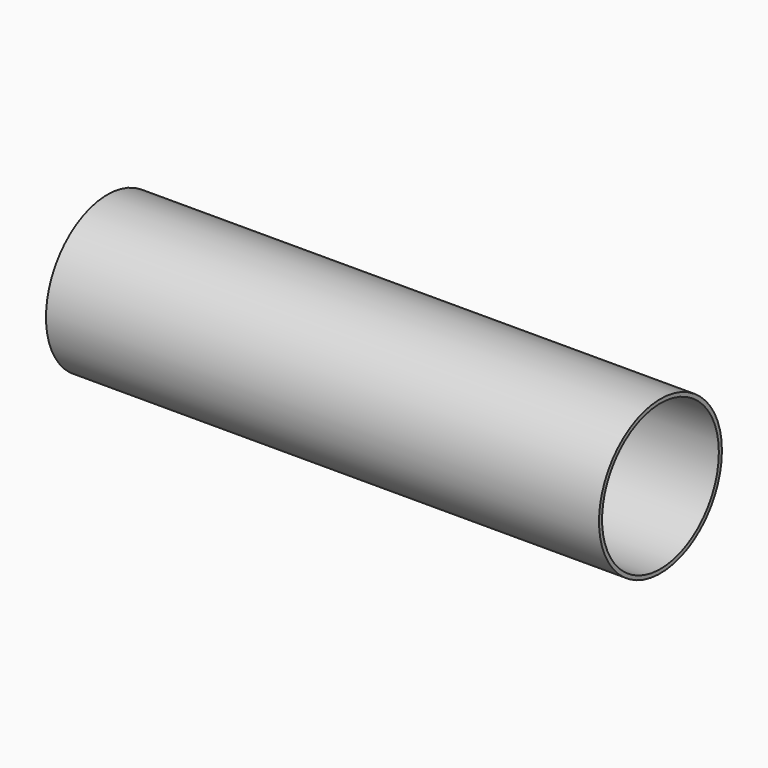
from build123d import *

# Parameters (mm, degrees)
F1_R     = 63.5
F1_R_2   = 60.325
F2_DEPTH = 457.2


# Not quite as in the source:
# - a variable given as a bare number and used for a length is read in inches; the dataset says mm whatever the document's units were


with BuildPart() as f2:
    # F1 (on Right) → F2 (new body)
    with BuildSketch(Plane.YZ):
        with Locations((13.9308627695, 20.094960928)):
            Circle(F1_R)
        with Locations((13.9308627695, 20.094960928)):
            Circle(F1_R_2, mode=Mode.SUBTRACT)
    extrude(amount=F2_DEPTH)


solid = f2.part
